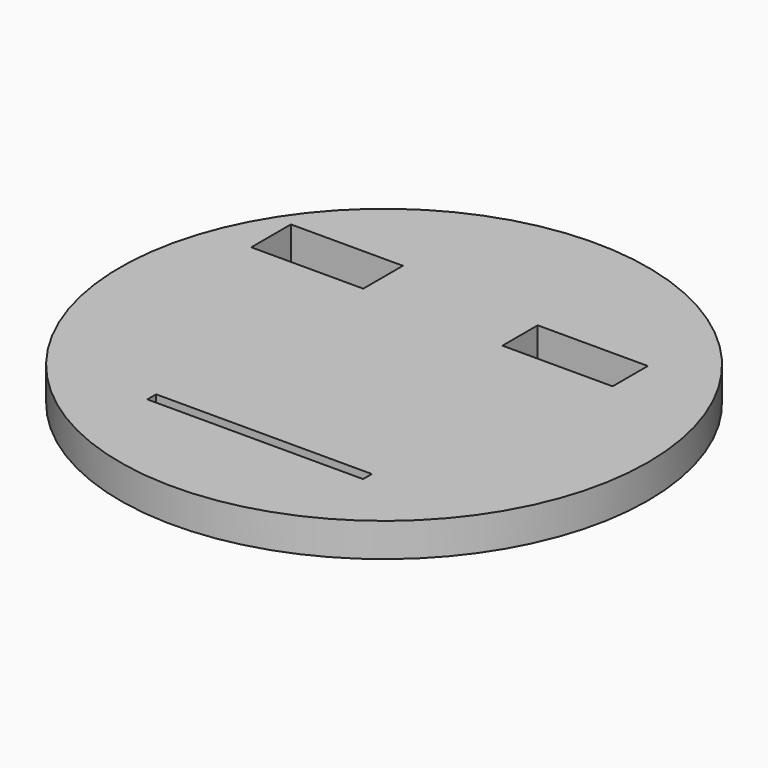
from build123d import *

# Parameters (mm, degrees)
F0_R     = 49.7916549323
F2_DEPTH = 6.35
F1_W     = 21.1281813681
F1_H     = 9.3518197536
F3_DEPTH = 6.351
F4_W     = 20.7818225026
F4_H     = 8.3127245307
F5_DEPTH = 6.351
F6_W     = 43.4686355293
F6_H     = 2.7709081769
F7_DEPTH = 145
F8_W     = 40.6977310777
F8_H     = 2.0781829953
F9_DEPTH = 6.351


# Not quite as in the source:
# - an extrude ends at something that could not be found from the text; its depth is read off the source's solid


with BuildPart() as f2:
    # F0 (on Top) → F2 (new body)
    with BuildSketch(Plane.XY):
        Circle(F0_R)
    extrude(amount=F2_DEPTH)

    # F1 (on face) → F3 (cut, through all)
    with BuildSketch(Plane.XY):
        with Locations((-28.1420461833, 21.7343177646)):
            Rectangle(F1_W, F1_H)
    extrude(amount=F3_DEPTH, mode=Mode.SUBTRACT)

    # F4 (on Top) → F5 (cut, through all)
    with BuildSketch(Plane.XY):
        with Locations((20.1756805182, 19.8293179274)):
            Rectangle(F4_W, F4_H)
    extrude(amount=F5_DEPTH, mode=Mode.SUBTRACT)

    # F6 (on face) → F7 (cut, through all)
    with BuildSketch(Plane.XY.offset(6.35)):
        with Locations((0, -21.9075009227)):
            Rectangle(F6_W, F6_H)
    extrude(amount=F7_DEPTH, mode=Mode.SUBTRACT)

    # F8 (on Top) → F9 (cut, through all)
    with BuildSketch(Plane.XY):
        with Locations((0, -29.3543189764)):
            Rectangle(F8_W, F8_H)
    extrude(amount=F9_DEPTH, mode=Mode.SUBTRACT)


solid = f2.part
